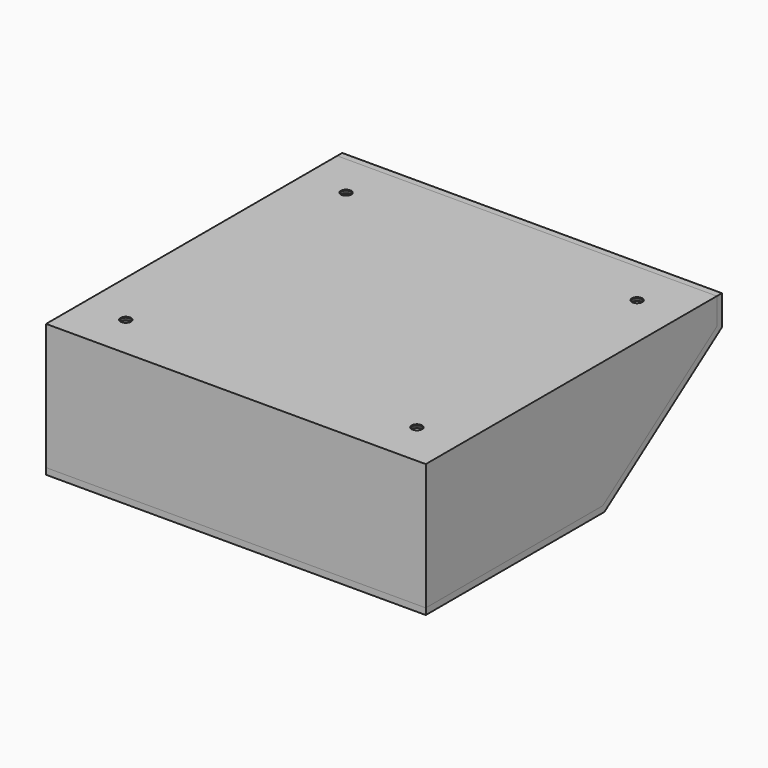
from build123d import *

# Parameters (mm, degrees)
F0_W             = 69.9466375641
F0_H             = 40
F1_DEPTH         = 120
F2_T             = -2
F3_W             = 7
F3_H             = 7
F4_DEPTH         = 38
F5_DEPTH         = 120
F6_W             = 73
F6_H             = 26
F6_R             = 3.5
F6_W_2           = 12
F6_H_2           = 20
F7_DEPTH         = 2
F9_D             = 2.5
F9_DEPTH         = 17.5
F9_CSINK_D       = 6.72
F9_CSINK_ANGLE   = 90
F9_TIP           = 0.7510757738
F9_2_D           = 2.5
F9_2_DEPTH       = 17.5
F9_2_CSINK_D     = 6.72
F9_2_CSINK_ANGLE = 90
F9_2_TIP         = 0.7510757738
F10_D            = 3.3
F10_DEPTH        = 25
F10_CSINK_D      = 6.72
F10_CSINK_ANGLE  = 90
F10_TIP          = 0.9914200214


with BuildPart() as f1:
    # F0 (on Right) → F1 (new body)
    with BuildSketch(Plane.YZ):
        with Locations((0, 20)):
            Rectangle(F0_W, F0_H)
        Polygon((34.9733187821, 40), (34.9733187821, 0), (80.0266812179, 31.5467039993), (80.0266812179, 40), align=None)
    extrude(amount=F1_DEPTH)

    # F2
    f2_openings = [f1.faces().sort_by_distance(p)[0] for p in [
        (60, 0, 0),
        (60, 57.5, 15.773352),
    ]]
    offset(amount=F2_T, openings=f2_openings)

    # F3 (on face) → F4 (join, through all)
    with BuildSketch(Plane(origin=(0, 0, 38), x_dir=(1, 0, 0), z_dir=(0, 0, -1))):
        with Locations((5.5, 29.4733187821)):
            Rectangle(F3_W, F3_H)
        with Locations((114.5, 29.4733187821)):
            Rectangle(F3_W, F3_H)
        with Locations((5.5, -28.5266812179)):
            Rectangle(F3_W, F3_H)
        with Locations((114.5, -28.5266812179)):
            Rectangle(F3_W, F3_H)
    extrude(amount=F4_DEPTH)

    # F9
    with Locations(Plane(origin=(0, 0, -2), x_dir=(1, 0, 0), z_dir=(0, 0, -1))):
        with Locations((114.5, -28.5266812179), (114.5, 29.4733187821), (5.5, 29.4733187821), (5.5, -28.5266812179)):
            CounterSinkHole(F9_D / 2, F9_CSINK_D / 2, depth=F9_DEPTH, counter_sink_angle=F9_CSINK_ANGLE)
            with Locations((0, 0, -(F9_DEPTH + F9_TIP / 2))):  # 118° drill point
                Cone(0, F9_D / 2, F9_TIP, mode=Mode.SUBTRACT)

    # F10
    with Locations(Plane(origin=(0, 0, 38), x_dir=(1, 0, 0), z_dir=(0, 0, -1))):
        with Locations((14, 20.9733187821), (106, 20.9733187821), (106, -66.0266812179), (14, -66.0266812179)):
            CounterSinkHole(F10_D / 2, F10_CSINK_D / 2, depth=F10_DEPTH, counter_sink_angle=F10_CSINK_ANGLE)
            with Locations((0, 0, -(F10_DEPTH + F10_TIP / 2))):  # 118° drill point
                Cone(0, F10_D / 2, F10_TIP, mode=Mode.SUBTRACT)


with BuildPart() as f5:
    # F0 (on Right) → F5 (new body, through all)
    with BuildSketch(Plane.YZ):
        Polygon((80.0266812179, 31.5467039993), (34.9733187821, 0), (-34.9733187821, 0), (-34.9733187821, -2), (35.6039163598, -2), (82.0266812179, 30.5055698982), (82.0266812179, 40), (80.0266812179, 40), align=None)
    extrude(amount=F5_DEPTH)

    # F6 (on face) → F7 (cut, through all)
    with BuildSketch(Plane(origin=(0, 12.6530225125, -18.0703888805), x_dir=(1, 0, 0), z_dir=(0, 0.5735764364, -0.8191520443))):
        with Locations((73, -56.3537338376)):
            Rectangle(F6_W, F6_H)
        with Locations((20, -42.0178679981)):
            Circle(F6_R)
        with Locations((20, -66.689599677)):
            Rectangle(F6_W_2, F6_H_2)
    extrude(amount=-F7_DEPTH, mode=Mode.SUBTRACT)

    # F9#2
    with Locations(Plane(origin=(0, 0, -2), x_dir=(1, 0, 0), z_dir=(0, 0, -1))):
        with Locations((114.5, -28.5266812179), (114.5, 29.4733187821), (5.5, 29.4733187821), (5.5, -28.5266812179)):
            CounterSinkHole(F9_2_D / 2, F9_2_CSINK_D / 2, depth=F9_2_DEPTH, counter_sink_angle=F9_2_CSINK_ANGLE)
            with Locations((0, 0, -(F9_2_DEPTH + F9_2_TIP / 2))):  # 118° drill point
                Cone(0, F9_2_D / 2, F9_2_TIP, mode=Mode.SUBTRACT)


solid = Compound([f1.part, f5.part])
